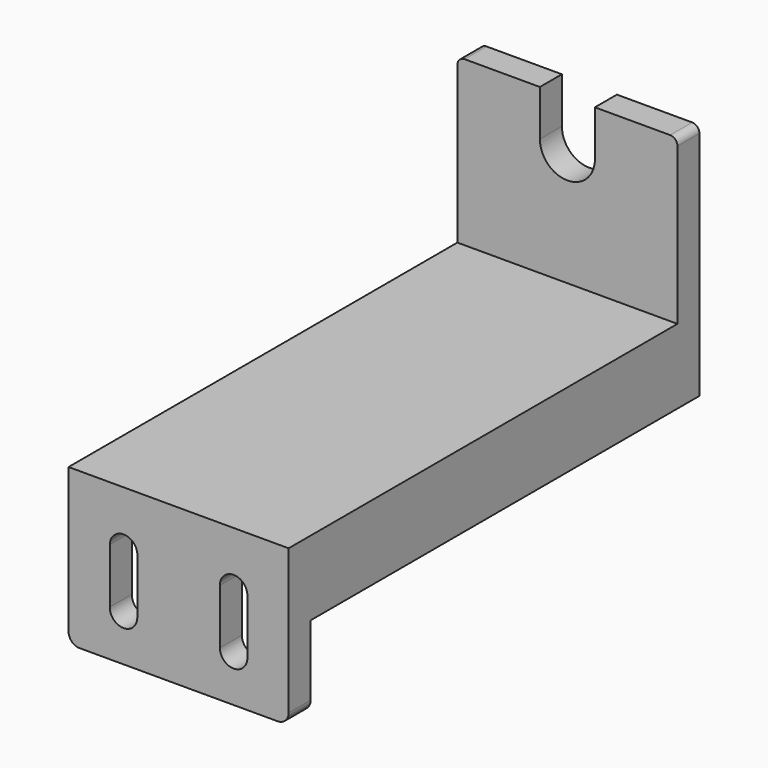
from build123d import *

# Parameters (mm, degrees)
F1_DEPTH = 317.5
F4_DEPTH = 19.05
F5_DEPTH = 19.05


# Not quite as in the source:
# - a feature names something its author has since deleted; it is built from what else it names


with BuildPart() as f1:
    # F0 (on Front) → F1 (new body)
    with BuildSketch(Plane.XZ):
        with BuildLine():
            Line((152.4, 0), (0, 0))
            Line((0, 0), (0, -51.6636))
            Line((0, -51.6636), (8.7122, -51.6636))
            Line((8.7122, -51.6636), (8.7122, -18.1356))
            ThreePointArc((8.7122, -18.1356), (11.6879951031, -10.9513951031), (18.8722, -7.9756))
            Line((18.8722, -7.9756), (133.5278, -7.9756))
            ThreePointArc((133.5278, -7.9756), (140.7120048969, -10.9513951031), (143.6878, -18.1356))
            Line((143.6878, -18.1356), (143.6878, -51.6636))
            Line((143.6878, -51.6636), (152.4, -51.6636))
            Line((152.4, -51.6636), (152.4, 0))
        make_face()
    extrude(amount=F1_DEPTH)

    # F3 (on face) → F4 (join)
    with BuildSketch(Plane(origin=(0, 0, 0), x_dir=(-1, 0, 0), z_dir=(0, 1, 0))):
        with BuildLine():
            Line((-152.4, 108.3564), (-152.4, 0))
            Line((-152.4, 0), (0, 0))
            Line((0, 0), (0, 108.3564))
            ThreePointArc((0, 108.3564), (-1.4878975516, 111.9485024484), (-5.08, 113.4364))
            Line((-5.08, 113.4364), (-57.15, 113.4364))
            Line((-57.15, 113.4364), (-57.15, 81.6864))
            ThreePointArc((-57.15, 81.6864), (-76.2, 62.6364), (-95.25, 81.6864))
            Line((-95.25, 81.6864), (-95.25, 113.4364))
            Line((-95.25, 113.4364), (-147.32, 113.4364))
            ThreePointArc((-147.32, 113.4364), (-150.9121024484, 111.9485024484), (-152.4, 108.3564))
        make_face()
        with BuildLine():
            Line((-143.6878, -18.1356), (-143.6878, -51.6636))
            Line((-143.6878, -51.6636), (-8.7122, -51.6636))
            Line((-8.7122, -51.6636), (-8.7122, -18.1356))
            ThreePointArc((-8.7122, -18.1356), (-11.6879951031, -10.9513951031), (-18.8722, -7.9756))
            Line((-18.8722, -7.9756), (-133.5278, -7.9756))
            ThreePointArc((-133.5278, -7.9756), (-140.7120048969, -10.9513951031), (-143.6878, -18.1356))
        make_face()
        with BuildLine():
            Line((-152.4, 0), (-152.4, -51.6636))
            Line((-152.4, -51.6636), (-143.6878, -51.6636))
            Line((-143.6878, -51.6636), (-143.6878, -18.1356))
            ThreePointArc((-143.6878, -18.1356), (-140.7120048969, -10.9513951031), (-133.5278, -7.9756))
            Line((-133.5278, -7.9756), (-18.8722, -7.9756))
            ThreePointArc((-18.8722, -7.9756), (-11.6879951031, -10.9513951031), (-8.7122, -18.1356))
            Line((-8.7122, -18.1356), (-8.7122, -51.6636))
            Line((-8.7122, -51.6636), (0, -51.6636))
            Line((0, -51.6636), (0, 0))
            Line((0, 0), (-152.4, 0))
        make_face()
    extrude(amount=F4_DEPTH)

    # F2 (on face) → F5 (join)
    with BuildSketch(Plane.XZ.offset(317.5)):
        with BuildLine():
            Line((152.4, 0), (0, 0))
            Line((0, 0), (0, -100.33))
            ThreePointArc((0, -100.33), (2.2318463274, -105.7181536726), (7.62, -107.95))
            Line((7.62, -107.95), (144.78, -107.95))
            ThreePointArc((144.78, -107.95), (150.1681536726, -105.7181536726), (152.4, -100.33))
            Line((152.4, -100.33), (152.4, 0))
        make_face()
        with BuildLine():
            Line((28.5572737867, -76.085673397), (28.5940985013, -37.985673397))
            ThreePointArc((28.5940985013, -37.985673397), (38.2314841006, -28.6802259255), (47.6427262133, -38.214326603))
            Line((47.6427262133, -38.214326603), (47.6059014987, -76.314326603))
            ThreePointArc((47.6059014987, -76.314326603), (37.9659922536, -85.8300138104), (28.5572737867, -76.085673397))
        make_face(mode=Mode.SUBTRACT)
        with BuildLine():
            Line((104.7750042372, -76.2000004751), (104.7749957628, -38.099982679))
            ThreePointArc((104.7749957628, -38.099982679), (114.3000041857, -28.5750016435), (123.8249957628, -38.0999995249))
            Line((123.8249957628, -38.0999995249), (123.8250042372, -76.200017321))
            ThreePointArc((123.8250042372, -76.200017321), (114.2999958142, -85.7250194396), (104.7750042372, -76.2000004751))
        make_face(mode=Mode.SUBTRACT)
    extrude(amount=F5_DEPTH)


solid = f1.part
